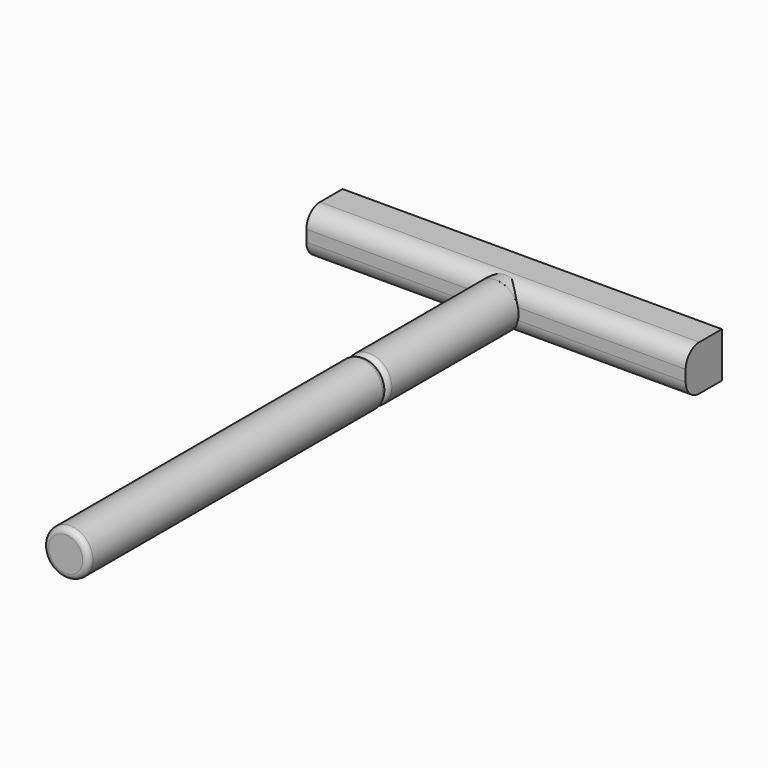
from build123d import *

# Parameters (mm, degrees)
F0_W     = 4
F0_H     = 29
F2_R     = 1
F0_H_2   = 2
F0_H_3   = 6
F3_DEPTH = 4
F5_R     = 0.99999
F6_R     = 1
F7_R     = 3


# Not quite as in the source:
# - a fillet or chamfer is up to 0.001 mm smaller than in the source, because OpenCascade refuses the exact size


with BuildPart() as f1:
    # F0 (on Top) → F1 (revolve)
    with BuildSketch(Plane.XY):
        with Locations((2, -18.5)):
            Rectangle(F0_W, F0_H)
    revolve(axis=Axis((0, -27.75, 0), (0, -1, 0)))

    # F2
    f2_edges = [f1.edges().sort_by_distance(p)[0] for p in [
        (-4, -33, 0),
    ]]
    fillet(f2_edges, radius=F2_R)

    # F0 (on Top) → F4 (revolve)
    with BuildSketch(Plane.XY):
        Polygon((4, -99), (4, -33), (0, -33), (0, -51.5), (0, -99), align=None)
    revolve(axis=Axis((0, -75.25, 0), (0, -1, 0)))

    # F5 (radius 1 in the source; OpenCascade refuses exactly that, so slightly less here)
    f5_edges = [f1.edges().sort_by_distance(p)[0] for p in [
        (-4, -33, 0),
    ]]
    fillet(f5_edges, radius=F5_R)

    # F6
    f6_edges = [f1.edges().sort_by_distance(p)[0] for p in [
        (-4, -99, 0),
    ]]
    fillet(f6_edges, radius=F6_R)


with BuildPart() as f3:
    # F0 (on Top) → F3 (new body, symmetric)
    with BuildSketch(Plane.XY):
        with Locations((2, -3)):
            Rectangle(F0_W, F0_H_2)
        with Locations((2, 1)):
            Rectangle(F0_W, F0_H_3)
        with Locations((-2, 1)):
            Rectangle(F0_W, F0_H_3)
        with Locations((-2, -3)):
            Rectangle(F0_W, F0_H_2)
        Polygon((33.5, -4), (33.5, 4), (4, 4), (4, -2), (4, -4), align=None)
        Polygon((-4, -2), (-4, 4), (-33.5, 4), (-33.5, -4), (-4, -4), align=None)
    extrude(amount=F3_DEPTH, both=True)

    # F7
    f7_edges = [f3.edges().sort_by_distance(p)[0] for p in [
        (0, -4, -4),
        (0, -4, 4),
    ]]
    fillet(f7_edges, radius=F7_R)


with BuildPart() as f8:
    # F0 (on Top) → F8 (revolve)
    with BuildSketch(Plane.XY):
        with Locations((-2, -3)):
            Rectangle(F0_W, F0_H_2)
    revolve(axis=Axis((0, 0, 0), (0, 1, 0)))


solid = Compound([f1.part, f3.part, f8.part])
